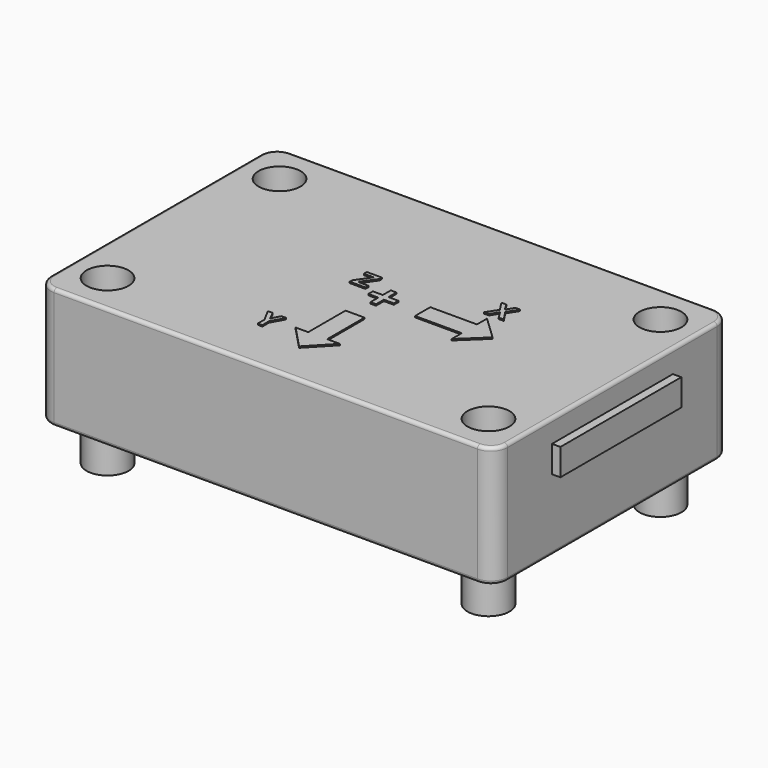
from build123d import *

# Parameters (mm, degrees)
F1_DEPTH       = 9.144
F2_R           = 0.254
F3_R           = 1.0033
F4_DEPTH       = 9.145
F5_R           = 1.5875
F6_DEPTH       = 1.8542
F7_W           = 11.4268660545
F7_H           = 2.0224535838
F8_DEPTH       = 0.635
F9_TEXT_SIZE   = 2.2291370745
F9_TEXT_SIZE_2 = 3.9707182118
F10_DEPTH      = 0.1
F11_R          = 1.5875
F11_R_2        = 0.8128
F12_DEPTH      = 3.175


# Not quite as in the source:
# - Text() gives the source's letters only with a copy of the font that has no kerning and outlines rounded to 1/6400 em; it was checked with that copy


with BuildPart() as f1:
    # F0 (on Top) → F1 (new body)
    with BuildSketch(Plane.XY):
        with BuildLine():
            Line((-16.002, -11.176), (16.002, -11.176))
            ThreePointArc((16.002, -11.176), (16.9000256121, -10.8040256121), (17.272, -9.906))
            Line((17.272, -9.906), (17.272, 9.906))
            ThreePointArc((17.272, 9.906), (16.9000256121, 10.8040256121), (16.002, 11.176))
            Line((16.002, 11.176), (-16.002, 11.176))
            ThreePointArc((-16.002, 11.176), (-16.9000256121, 10.8040256121), (-17.272, 9.906))
            Line((-17.272, 9.906), (-17.272, -9.906))
            ThreePointArc((-17.272, -9.906), (-16.9000256121, -10.8040256121), (-16.002, -11.176))
        make_face()
    extrude(amount=F1_DEPTH)

    # F2
    f2_edges = [f1.edges().sort_by_distance(p)[0] for p in [
        (0, -11.176, 9.144),
        (0, -11.176, 0),
        (16.900026, -10.804026, 0),
        (17.272, 0, 0),
        (16.900026, 10.804026, 0),
        (0, 11.176, 0),
        (-16.900026, 10.804026, 0),
        (-17.272, 0, 0),
        (-16.900026, -10.804026, 0),
    ]]
    fillet(f2_edges, radius=F2_R)

    # F3 (on face) → F4 (cut, through all)
    with BuildSketch(Plane.XY.offset(9.144)):
        with Locations((-14.4018, 8.128)):
            Circle(F3_R)
        with Locations((14.4018, 8.128)):
            Circle(F3_R)
        with Locations((-14.4018, -8.128)):
            Circle(F3_R)
        with Locations((14.4018, -8.128)):
            Circle(F3_R)
    extrude(amount=-F4_DEPTH, mode=Mode.SUBTRACT)

    # F5 (on face) → F6 (cut)
    with BuildSketch(Plane.XY.offset(9.144)):
        with Locations((-14.4018, 8.128)):
            Circle(F5_R)
        with Locations((14.4018, 8.128)):
            Circle(F5_R)
        with Locations((14.4018, -8.128)):
            Circle(F5_R)
        with Locations((-14.4018, -8.128)):
            Circle(F5_R)
    extrude(amount=-F6_DEPTH, mode=Mode.SUBTRACT)


with BuildPart() as f8:
    # F7 (on face) → F8 (new body)
    with BuildSketch(Plane.YZ.offset(17.272)):
        with Locations((0, 6.4174896106)):
            Rectangle(F7_W, F7_H)
    extrude(amount=F8_DEPTH)


with BuildPart() as f10:
    # F9 (on face) → F10 (new body)
    with BuildSketch(Plane.XY.offset(9.144)):
        Polygon((2.9211144429, 0.7217947859), (2.9211144429, 0.0048919118), (2.9211144429, -0.7120109624), (6.4491813537, -0.7120109624), (6.4491813537, -1.6648031999), (8.2060957503, 0.0048919118), (6.4491813537, 1.6745870234), (6.4491813537, 0.7217947859), align=None)
        Polygon((0.7217947859, -2.746458631), (0.0048919118, -2.746458631), (-0.7120109624, -2.746458631), (-0.7120109624, -6.2745255418), (-1.6648031999, -6.2745255418), (0.0048919118, -8.0314399384), (1.6745870234, -6.2745255418), (0.7217947859, -6.2745255418), align=None)
        with Locations((5.8073883411, 2.2055885056)):
            Text('X', F9_TEXT_SIZE, font='Open Sans', font_style=FontStyle.BOLD, text_align=(TextAlign.LEFT, TextAlign.BOTTOM))
        with Locations((-4.2545874603, -7.2545250878)):
            Text('Y', F9_TEXT_SIZE, font='Open Sans', font_style=FontStyle.BOLD, text_align=(TextAlign.LEFT, TextAlign.BOTTOM))
        with Locations((-2.8853494441, 0.3014651593)):
            Text('Z', F9_TEXT_SIZE, font='Open Sans', font_style=FontStyle.BOLD, text_align=(TextAlign.LEFT, TextAlign.BOTTOM))
        with Locations((-1.1623183964, -1.4240783639)):
            Text('+', F9_TEXT_SIZE_2, font='Open Sans', font_style=FontStyle.BOLD, text_align=(TextAlign.LEFT, TextAlign.BOTTOM))
    extrude(amount=F10_DEPTH)


with BuildPart() as f12:
    # F11 (on face) → F12 (new body)
    with BuildSketch(Plane(origin=(0, 0, 0), x_dir=(1, 0, 0), z_dir=(0, 0, -1))):
        with Locations((-14.4018, 8.128)):
            Circle(F11_R)
        with Locations((-14.4018, 8.128)):
            Circle(F11_R_2, mode=Mode.SUBTRACT)
    extrude(amount=F12_DEPTH)


with BuildPart() as f12b:
    # F11 (on face) → F12, piece 2 (new body)
    with BuildSketch(Plane(origin=(0, 0, 0), x_dir=(1, 0, 0), z_dir=(0, 0, -1))):
        with Locations((14.4018, 8.128)):
            Circle(F11_R)
        with Locations((14.4018, 8.128)):
            Circle(F11_R_2, mode=Mode.SUBTRACT)
    extrude(amount=F12_DEPTH)


with BuildPart() as f12c:
    # F11 (on face) → F12, piece 3 (new body)
    with BuildSketch(Plane(origin=(0, 0, 0), x_dir=(1, 0, 0), z_dir=(0, 0, -1))):
        with Locations((-14.4018, -8.128)):
            Circle(F11_R)
        with Locations((-14.4018, -8.128)):
            Circle(F11_R_2, mode=Mode.SUBTRACT)
    extrude(amount=F12_DEPTH)


with BuildPart() as f12d:
    # F11 (on face) → F12, piece 4 (new body)
    with BuildSketch(Plane(origin=(0, 0, 0), x_dir=(1, 0, 0), z_dir=(0, 0, -1))):
        with Locations((14.4018, -8.128)):
            Circle(F11_R)
        with Locations((14.4018, -8.128)):
            Circle(F11_R_2, mode=Mode.SUBTRACT)
    extrude(amount=F12_DEPTH)


solid = Compound([f1.part, f8.part, f10.part, f12.part, f12b.part, f12c.part, f12d.part])
